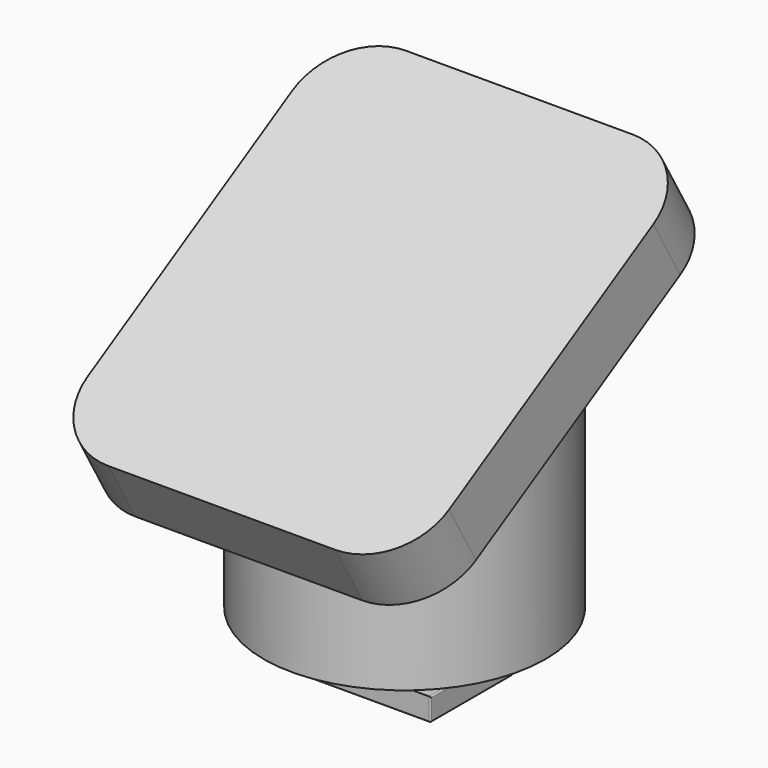
from build123d import *

# Parameters (mm, degrees)
F0_W           = 1
F0_H           = 2.65
F0_H_2         = 2.4
F0_W_2         = 9
F1_DEPTH       = 1.7
F2_DEPTH       = 4.3
F3_START       = 2.6
F3_DEPTH       = 1.7
F4_DEPTH       = 2.6
F5_START       = 0.1
F0_R           = 10.5
F5_DEPTH       = 1.6
F6_R           = 0.09999
F7_R           = 10.5
F8_DEPTH       = 22
F10_DEPTH      = 39.6047188237
F10_DEPTH_BACK = 25
F11_R          = 4.05
F12_DEPTH      = 3.07
F13_W          = 26.8920833189
F13_H          = 31.9528504953
F14_DEPTH      = 5
F13_R          = 4.05
F15_DEPTH      = 3.05
F16_START      = 3.05
F16_DEPTH      = 1.95
F17_R          = 5


# Not quite as in the source:
# - a fillet or chamfer is up to 0.001 mm smaller than in the source, because OpenCascade refuses the exact size


with BuildPart() as f1:
    # F0 (on Top) → F1 (new body)
    with BuildSketch(Plane.XY):
        with Locations((-33.6037188237, 9.8102559388)):
            Rectangle(F0_W, F0_H)
        with Locations((-33.6037188237, 7.2852559388)):
            Rectangle(F0_W, F0_H_2)
        with Locations((-28.6037188237, 9.8102559388)):
            Rectangle(F0_W_2, F0_H)
        with Locations((-28.6037188237, 7.2852559388)):
            Rectangle(F0_W_2, F0_H_2)
        with Locations((-28.6037188237, 4.7602559388)):
            Rectangle(F0_W_2, F0_H)
        with Locations((-33.6037188237, 4.7602559388)):
            Rectangle(F0_W, F0_H)
    extrude(amount=F1_DEPTH)

    # F0 (on Top) → F2 (join)
    with BuildSketch(Plane.XY):
        with Locations((-28.6037188237, 7.2852559388)):
            Rectangle(F0_W_2, F0_H_2)
    extrude(amount=-F2_DEPTH)

    # F1_face (on face) → F3 (join)
    with BuildSketch(Plane(origin=(-29.298664672, 7.2852559388, 0), x_dir=(1, 0, 0), z_dir=(0, 0, -1)).offset(F3_START)):
        Polygon((-4.8050541516, -3.85), (5.1949458484, -3.85), (5.1949458484, -1.2), (-3.8050541516, -1.2), (-3.8050541516, 1.2), (5.1949458484, 1.2), (5.1949458484, 3.85), (-4.8050541516, 3.85), align=None)
    extrude(amount=F3_DEPTH)

    # F0 (on Top) → F4 (join, through all)
    with BuildSketch(Plane.XY):
        with Locations((-33.6037188237, 9.8102559388)):
            Rectangle(F0_W, F0_H)
        with Locations((-33.6037188237, 7.2852559388)):
            Rectangle(F0_W, F0_H_2)
        with Locations((-33.6037188237, 4.7602559388)):
            Rectangle(F0_W, F0_H)
    extrude(amount=-F4_DEPTH)

    # F0 (on Top) → F5 (join)
    with BuildSketch(Plane.XY.offset(F5_START)):
        with Locations((-29.1037188237, 7.2852559388)):
            Circle(F0_R)
        Polygon((-34.1037188237, 8.4852559388), (-34.1037188237, 11.1352559388), (-33.1037188237, 11.1352559388), (-24.1037188237, 11.1352559388), (-24.1037188237, 8.4852559388), (-24.1037188237, 6.0852559388), (-24.1037188237, 3.4352559388), (-33.1037188237, 3.4352559388), (-34.1037188237, 3.4352559388), (-34.1037188237, 6.0852559388), align=None, mode=Mode.SUBTRACT)
    extrude(amount=F5_DEPTH)

    # F6 (radius 0.1 in the source; OpenCascade refuses exactly that, so slightly less here)
    f6_edges = [f1.edges().sort_by_distance(p)[0] for p in [
        (-24.103719, 4.760256, 0),
        (-24.103719, 9.810256, 0),
        (-24.103719, 6.085256, -1.3),
        (-24.103719, 8.485256, -1.3),
        (-24.103719, 9.810256, -2.6),
        (-24.103719, 4.760256, -2.6),
        (-24.103719, 3.435256, -3.45),
        (-24.103719, 7.285256, -4.3),
        (-24.103719, 11.135256, -3.45),
        (-28.603719, 3.435256, 0),
        (-28.603719, 11.135256, 0),
        (-29.103719, 3.435256, -4.3),
        (-29.103719, 11.135256, -4.3),
    ]]
    fillet(f6_edges, radius=F6_R)

    # F7 (on face) → F8 (join)
    with BuildSketch(Plane.XY.offset(1.7)):
        with Locations((-29.1037188237, 7.2852559388)):
            Circle(F7_R)
    extrude(amount=F8_DEPTH)

    # F9 (on Right) → F10 (cut, two sides)
    with BuildSketch(Plane.YZ) as f10_sk:
        Polygon((17.7852559388, 23.7), (-3.2147440612, 23.7), (-7.2555868058, 9.2426627007), (-1.8645326524, 12.3551892673), align=None)
    extrude(amount=-F10_DEPTH, mode=Mode.SUBTRACT)
    extrude(f10_sk.sketch, amount=F10_DEPTH_BACK, mode=Mode.SUBTRACT)

    # F11 (on face) → F12 (cut)
    with BuildSketch(Plane(origin=(0, -5.8160870502, 10.0737582721), x_dir=(1, 0, 0), z_dir=(0, -0.5, 0.8660254038))):
        with Locations((-29.1037188237, 9.5081278028)):
            Circle(F11_R)
        with Locations((-29.1037188237, 20.7481278028)):
            Circle(F11_R)
    extrude(amount=-F12_DEPTH, mode=Mode.SUBTRACT)


with BuildPart() as f14:
    # F13 (on face) → F14 (new body)
    with BuildSketch(Plane(origin=(0, -5.8160870502, 10.0737582721), x_dir=(1, 0, 0), z_dir=(0, -0.5, 0.8660254038))):
        with Locations((-29.0497604831, 14.2760582082)):
            Rectangle(F13_W, F13_H)
        with BuildLine():
            Line((-18.6037188237, 1.2996329605), (-39.4958021426, 1.2996329605))
            Line((-39.4958021426, 1.2996329605), (-39.4958021426, 13.2724569986))
            add(Edge.make_bspline(
                [(-39.6037188237, 15.1281280197), (-39.6037188363, 14.1954998359), (-39.4958021426, 13.2724569986)],
                knots=[4.7123889637, 4.7123889637, 4.7123889637, 4.8674305263, 4.8674305263, 4.8674305263], degree=2, weights=[1, 0.9710906997, 0.9478882411]))
            add(Edge.make_bspline(
                [(-39.4958021426, 16.983798607), (-39.603718811, 16.0607559855), (-39.6037188237, 15.1281280197)],
                knots=[4.5573474366, 4.5573474366, 4.5573474366, 4.7123889637, 4.7123889637, 4.7123889637], degree=2, weights=[0.9478882526, 0.9710907067, 1]))
            Line((-39.4958021426, 16.983798607), (-39.4958021426, 27.2524834558))
            Line((-39.4958021426, 27.2524834558), (-32.8458187492, 27.2524834558))
            add(Edge.make_bspline(
                [(-25.3616188981, 27.2524834558), (-27.1691542693, 28.1045530304), (-29.1037187359, 28.1045530504), (-31.0382832932, 28.1045530704), (-32.8458187492, 27.2524834558)],
                knots=[2.7613255041, 2.7613255041, 2.7613255041, 3.1415926452, 3.1415926452, 3.521859803, 3.521859803, 3.521859803], degree=2, weights=[0.8925198158, 0.9290947753, 1, 0.9290947722, 0.8925198127]))
            Line((-25.3616188981, 27.2524834558), (-18.6037188237, 27.2524834558))
            Line((-18.6037188237, 27.2524834558), (-18.6037188237, 15.1281278028))
            Line((-18.6037188237, 15.1281278028), (-18.6037188237, 1.2996329605))
        make_face(mode=Mode.SUBTRACT)
        with BuildLine():
            Line((-39.4958021426, 13.2724569986), (-39.4958021426, 1.2996329605))
            Line((-39.4958021426, 1.2996329605), (-18.6037188237, 1.2996329605))
            Line((-18.6037188237, 1.2996329605), (-18.6037188237, 15.1281278028))
            add(Edge.make_bspline(
                [(-29.1037188237, 2.1517025552), (-18.6037188237, 2.1517025552), (-18.6037188237, 15.1281278028)],
                knots=[0, 0, 0, 1.5707963268, 1.5707963268, 1.5707963268], degree=2, weights=[1, 0.7071067812, 1]))
            add(Edge.make_bspline(
                [(-39.4958021426, 13.2724569986), (-38.1956294939, 2.1517025552), (-29.1037188237, 2.1517025552)],
                knots=[4.8674305263, 4.8674305263, 4.8674305263, 6.2831853072, 6.2831853072, 6.2831853072], degree=2, weights=[0.9478882411, 0.7360160756, 1]))
        make_face()
        with BuildLine():
            add(Edge.make_bspline(
                [(-18.6037188237, 15.1281278028), (-18.6037188237, 24.0668190788), (-25.3616188981, 27.2524834558)],
                knots=[1.5707963268, 1.5707963268, 1.5707963268, 2.7613255041, 2.7613255041, 2.7613255041], degree=2, weights=[1, 0.7780120088, 0.8925198158]))
            Line((-18.6037188237, 15.1281278028), (-18.6037188237, 27.2524834558))
            Line((-18.6037188237, 27.2524834558), (-25.3616188981, 27.2524834558))
        make_face()
        with BuildLine():
            Line((-39.4958021426, 27.2524834558), (-39.4958021426, 16.983798607))
            add(Edge.make_bspline(
                [(-32.8458187492, 27.2524834558), (-38.6131013788, 24.5337947178), (-39.4958021426, 16.983798607)],
                knots=[3.521859803, 3.521859803, 3.521859803, 4.5573474366, 4.5573474366, 4.5573474366], degree=2, weights=[0.8925198127, 0.7929242584, 0.9478882526]))
            Line((-32.8458187492, 27.2524834558), (-39.4958021426, 27.2524834558))
        make_face()
    extrude(amount=F14_DEPTH)

    # F13 (on face) → F14, piece 2 (join)
    with BuildSketch(Plane(origin=(0, -5.8160870502, 10.0737582721), x_dir=(1, 0, 0), z_dir=(0, -0.5, 0.8660254038))):
        with BuildLine():
            add(Edge.make_bspline(
                [(-18.6037188237, 15.1281278028), (-18.6037188237, -14.1426560497), (-36.5283400261, 6.5549137031), (-38.9966235925, 9.4050420661), (-39.4958021426, 13.394305708)],
                knots=[4.7123889804, 4.7123889804, 4.7123889804, 7.0685834706, 7.0685834706, 7.7623255267, 7.7623255267, 7.7623255267], degree=2, weights=[1, 0.3826834324, 1, 0.8182414624, 0.7435144471]))
            add(Edge.make_bspline(
                [(-29.1037188237, 27.2524834558), (-18.6037188237, 27.2524834558), (-18.6037188237, 15.1281278028)],
                knots=[3.1415926536, 3.1415926536, 3.1415926536, 4.7123889804, 4.7123889804, 4.7123889804], degree=2, weights=[1, 0.7071067812, 1]))
            add(Edge.make_bspline(
                [(-39.4958021426, 16.8619498976), (-38.1956294939, 27.2524834558), (-29.1037188237, 27.2524834558)],
                knots=[8.0258450855, 8.0258450855, 8.0258450855, 9.4247779608, 9.4247779608, 9.4247779608], degree=2, weights=[0.7021873252, 0.6334833799, 1]))
            Line((-39.4958021426, 16.8619498976), (-39.4958021426, 13.394305708))
        make_face()
        with Locations((-29.1037188237, 9.5081278028)):
            Circle(F13_R, mode=Mode.SUBTRACT)
        with Locations((-29.1037188237, 20.7481278028)):
            Circle(F13_R, mode=Mode.SUBTRACT)
        with BuildLine():
            add(Edge.make_bspline(
                [(-39.4958021426, 13.394305708), (-39.6037188372, 14.2567388914), (-39.6037188237, 15.1281280197)],
                knots=[7.7623255267, 7.7623255267, 7.7623255267, 7.8959689632, 7.8959689632, 7.8959689632], degree=2, weights=[0.7435144471, 0.7291189307, 0.7186954298]))
            Line((-39.4958021426, 13.394305708), (-39.4958021426, 16.8619498976))
            add(Edge.make_bspline(
                [(-39.6037188237, 15.1281280197), (-39.6037188102, 15.99951693), (-39.4958021426, 16.8619498976)],
                knots=[7.8959689632, 7.8959689632, 7.8959689632, 8.0258450855, 8.0258450855, 8.0258450855], degree=2, weights=[0.7186954298, 0.70856576, 0.7021873252]))
        make_face()
    extrude(amount=F14_DEPTH)

    # F11 (on face) → F15 (join)
    with BuildSketch(Plane(origin=(0, -5.8160870502, 10.0737582721), x_dir=(1, 0, 0), z_dir=(0, -0.5, 0.8660254038))):
        with BuildLine():
            add(Edge.make_bspline(
                [(-29.1037188237, 27.2524834558), (-18.6037188237, 27.2524834558), (-18.6037188237, 15.1281278028)],
                knots=[3.1415926536, 3.1415926536, 3.1415926536, 4.7123889804, 4.7123889804, 4.7123889804], degree=2, weights=[1, 0.7071067812, 1]))
            add(Edge.make_bspline(
                [(-18.6037188237, 15.1281278028), (-18.6037188237, 28.104552942), (-29.1037187359, 28.1045530504), (-39.6037186481, 28.1045531589), (-39.6037188237, 15.1281280197)],
                knots=[1.5707963268, 1.5707963268, 1.5707963268, 3.1415926452, 3.1415926452, 4.7123889637, 4.7123889637, 4.7123889637], degree=2, weights=[1, 0.7071067841, 1, 0.7071067841, 1]))
            add(Edge.make_bspline(
                [(-39.6037188237, 15.1281280197), (-39.6037186358, 27.2524834558), (-29.1037188237, 27.2524834558)],
                knots=[7.8959689632, 7.8959689632, 7.8959689632, 9.4247779608, 9.4247779608, 9.4247779608], degree=2, weights=[0.7186954298, 0.599456188, 1]))
        make_face()
        with BuildLine():
            add(Edge.make_bspline(
                [(-39.6037188237, 15.1281280197), (-39.6037189992, 2.1517025552), (-29.1037188237, 2.1517025552)],
                knots=[4.7123889637, 4.7123889637, 4.7123889637, 6.2831853072, 6.2831853072, 6.2831853072], degree=2, weights=[1, 0.7071067753, 1]))
            add(Edge.make_bspline(
                [(-29.1037188237, 2.1517025552), (-18.6037188237, 2.1517025552), (-18.6037188237, 15.1281278028)],
                knots=[0, 0, 0, 1.5707963268, 1.5707963268, 1.5707963268], degree=2, weights=[1, 0.7071067812, 1]))
            add(Edge.make_bspline(
                [(-18.6037188237, 15.1281278028), (-18.6037188237, -14.1426560497), (-36.5283400261, 6.5549137031), (-39.6037189015, 10.1060553462), (-39.6037188237, 15.1281280197)],
                knots=[4.7123889804, 4.7123889804, 4.7123889804, 7.0685834706, 7.0685834706, 7.8959689632, 7.8959689632, 7.8959689632], degree=2, weights=[1, 0.3826834324, 1, 0.7832272444, 0.7186954298]))
        make_face()
    extrude(amount=F15_DEPTH)

    # F11 (on face) → F16 (join)
    with BuildSketch(Plane(origin=(0, -5.8160870502, 10.0737582721), x_dir=(1, 0, 0), z_dir=(0, -0.5, 0.8660254038)).offset(F16_START)):
        with Locations((-29.1037188237, 20.7481278028)):
            Circle(F11_R)
        with Locations((-29.1037188237, 9.5081278028)):
            Circle(F11_R)
        with BuildLine():
            add(Edge.make_bspline(
                [(-29.1037188237, 27.2524834558), (-18.6037188237, 27.2524834558), (-18.6037188237, 15.1281278028)],
                knots=[3.1415926536, 3.1415926536, 3.1415926536, 4.7123889804, 4.7123889804, 4.7123889804], degree=2, weights=[1, 0.7071067812, 1]))
            add(Edge.make_bspline(
                [(-18.6037188237, 15.1281278028), (-18.6037188237, 28.104552942), (-29.1037187359, 28.1045530504), (-39.6037186481, 28.1045531589), (-39.6037188237, 15.1281280197)],
                knots=[1.5707963268, 1.5707963268, 1.5707963268, 3.1415926452, 3.1415926452, 4.7123889637, 4.7123889637, 4.7123889637], degree=2, weights=[1, 0.7071067841, 1, 0.7071067841, 1]))
            add(Edge.make_bspline(
                [(-39.6037188237, 15.1281280197), (-39.6037186358, 27.2524834558), (-29.1037188237, 27.2524834558)],
                knots=[7.8959689632, 7.8959689632, 7.8959689632, 9.4247779608, 9.4247779608, 9.4247779608], degree=2, weights=[0.7186954298, 0.599456188, 1]))
        make_face()
        with BuildLine():
            add(Edge.make_bspline(
                [(-39.6037188237, 15.1281280197), (-39.6037189992, 2.1517025552), (-29.1037188237, 2.1517025552)],
                knots=[4.7123889637, 4.7123889637, 4.7123889637, 6.2831853072, 6.2831853072, 6.2831853072], degree=2, weights=[1, 0.7071067753, 1]))
            add(Edge.make_bspline(
                [(-29.1037188237, 2.1517025552), (-18.6037188237, 2.1517025552), (-18.6037188237, 15.1281278028)],
                knots=[0, 0, 0, 1.5707963268, 1.5707963268, 1.5707963268], degree=2, weights=[1, 0.7071067812, 1]))
            add(Edge.make_bspline(
                [(-18.6037188237, 15.1281278028), (-18.6037188237, -14.1426560497), (-36.5283400261, 6.5549137031), (-39.6037189015, 10.1060553462), (-39.6037188237, 15.1281280197)],
                knots=[4.7123889804, 4.7123889804, 4.7123889804, 7.0685834706, 7.0685834706, 7.8959689632, 7.8959689632, 7.8959689632], degree=2, weights=[1, 0.3826834324, 1, 0.7832272444, 0.7186954298]))
        make_face()
    extrude(amount=F16_DEPTH)

    # F17
    f17_edges = [f14.edges().sort_by_distance(p)[0] for p in [
        (-42.495802, -8.538648, 11.388638),
        (-42.495802, 19.133332, 27.365064),
        (-15.603719, 19.133332, 27.365064),
        (-15.603719, -8.538648, 11.388638),
    ]]
    fillet(f17_edges, radius=F17_R)


solid = Compound([f1.part, f14.part])
